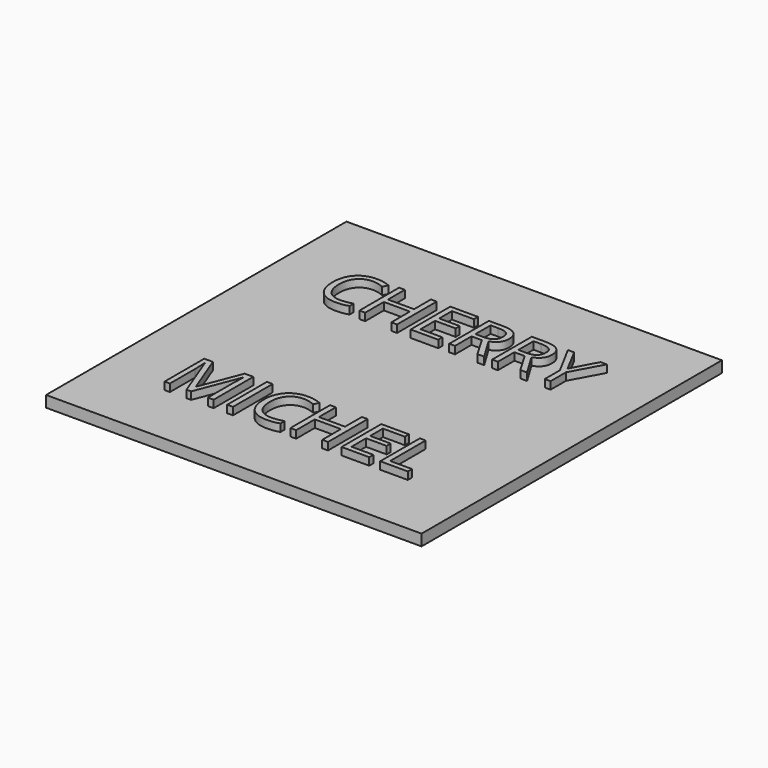
from build123d import *

# Parameters (mm, degrees)
F0_W         = 50
F0_H         = 50
F1_DEPTH     = 1.5
F2_TEXT_SIZE = 9.2447379282
F3_DEPTH     = 1


# Not quite as in the source:
# - Text() gives the source's letters only with a copy of the font that has no kerning and outlines rounded to 1/6400 em; it was checked with that copy


with BuildPart() as f1:
    # F0 (on Top) → F1 (new body)
    with BuildSketch(Plane.XY):
        Rectangle(F0_W, F0_H)
    extrude(amount=F1_DEPTH)

    # F2 (on face) → F3 (join)
    with BuildSketch(Plane.XY.offset(1.5)):
        with Locations((-16.968312806, 8.6929916888)):
            Text('CHERRY', F2_TEXT_SIZE, font='Open Sans', text_align=(TextAlign.LEFT, TextAlign.BOTTOM))
        with Locations((-16.968312806, -16.4526954758)):
            Text('MICHEL', F2_TEXT_SIZE, font='Open Sans', text_align=(TextAlign.LEFT, TextAlign.BOTTOM))
    extrude(amount=F3_DEPTH)


solid = f1.part
